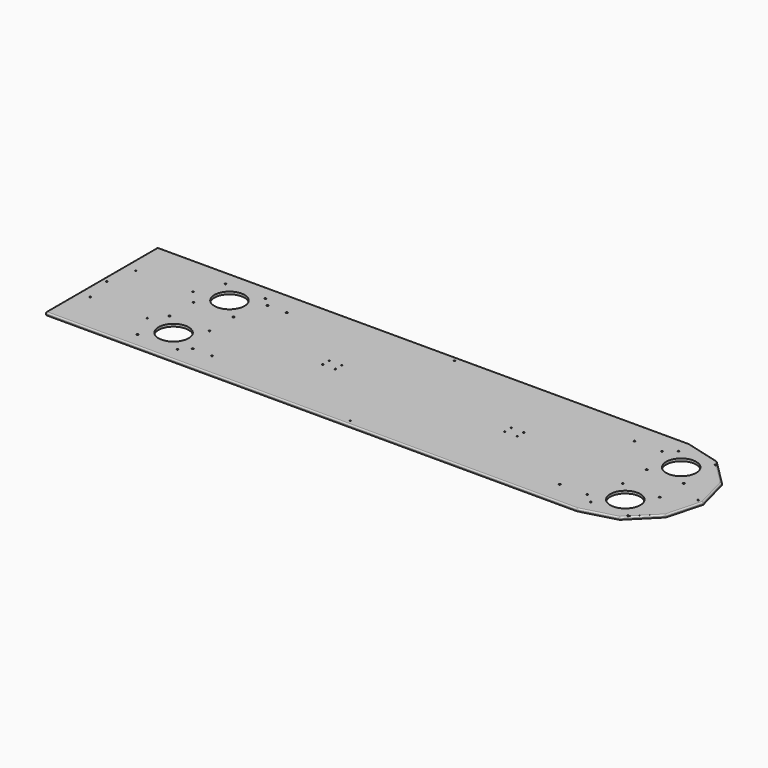
from build123d import *

# Parameters (mm, degrees)
F0_R         = 1.7272
F1_DEPTH     = 6.35
F2_R         = 1.7272
F2_R_2       = 38.1
F2_R_3       = 2.15265
F3_DEPTH     = 6.35
F4_R         = 1.7272
F4_R_2       = 2.15265
F5_DEPTH     = 6.35
F6_R         = 3.96875
F7_T1_DEPTH  = 90.4501332312
F7_T3_DEPTH  = 89.9092057235
F7_T5_DEPTH  = 1341.7087541502
F7_T7_DEPTH  = 89.9092057235
F7_T9_DEPTH  = 347.6625
F7_T11_DEPTH = 89.9092057235
F7_T13_DEPTH = 89.9092057235
F7_T15_DEPTH = 90.4501332312
F7_T18_ANGLE = 90
F7_T20_ANGLE = 30
F7_T22_ANGLE = 15
F7_T24_ANGLE = 30
F7_T26_ANGLE = 90
F7_T28_ANGLE = 30
F7_T30_ANGLE = 30
F7_T32_ANGLE = 15
F7_T34_ANGLE = 30


# Not quite as in the source:
# - a fillet or chamfer that OpenCascade refuses, or shapes differently, is made with other operations: its cross-section is extruded or revolved along the edge and cut away or added


with BuildPart() as f1:
    # F0 (on Top) → F1 (new body)
    with BuildSketch(Plane.XY):
        Polygon((88.9, 153.9793167929), (0, 177.8), (-1346.2, 177.8), (-1346.2, -177.8), (0, -177.8), (88.9, -153.9793167929), (153.9793167929, -88.9), (177.8, 0), (153.9793167929, 88.9), align=None)
        with Locations((-1316.83125, -72.23125)):
            Circle(F0_R, mode=Mode.SUBTRACT)
        with Locations((-1172.36875, -72.23125)):
            Circle(F0_R, mode=Mode.SUBTRACT)
        with Locations((-1316.83125, 72.23125)):
            Circle(F0_R, mode=Mode.SUBTRACT)
        with Locations((-1172.36875, 72.23125)):
            Circle(F0_R, mode=Mode.SUBTRACT)
    extrude(amount=F1_DEPTH)

    # F2 (on face) → F3 (cut, through all)
    with BuildSketch(Plane.XY.offset(6.35)):
        with Locations((-1333.0519925088, 0)):
            Circle(F2_R)
        with Locations((-584.2, 164.6519925088)):
            Circle(F2_R)
        with Locations((-584.2, -164.6519925088)):
            Circle(F2_R)
        with Locations((164.6519925088, 0)):
            Circle(F2_R)
        with Locations((51.0994784628, 88.5068929378)):
            Circle(F2_R_2)
        with Locations((51.0994784628, -88.5068929378)):
            Circle(F2_R_2)
        with Locations((-1092.835, 88.5068929378)):
            Circle(F2_R_2)
        with Locations((-1092.835, -88.5068929378)):
            Circle(F2_R_2)
        with Locations((4.1340214009, -139.1330868203)):
            Circle(F2_R_3)
        with Locations((98.0649355247, -139.1330868203)):
            Circle(F2_R_3)
        with Locations((98.0649355247, -37.8806990553)):
            Circle(F2_R_3)
        with Locations((4.1340214009, -37.8806990553)):
            Circle(F2_R_3)
        with Locations((4.1340214009, 37.8806990553)):
            Circle(F2_R_3)
        with Locations((4.1340214009, 139.1330868203)):
            Circle(F2_R_3)
        with Locations((98.0649355247, 139.1330868203)):
            Circle(F2_R_3)
        with Locations((98.0649355247, 37.8806990553)):
            Circle(F2_R_3)
        with Locations((-1143.4611938825, -139.1330868203)):
            Circle(F2_R_3)
        with Locations((-1042.2088061175, -139.1330868203)):
            Circle(F2_R_3)
        with Locations((-1042.2088061175, -37.8806990553)):
            Circle(F2_R_3)
        with Locations((-1143.4611938825, -37.8806990553)):
            Circle(F2_R_3)
        with Locations((-1143.4611938825, 37.8806990553)):
            Circle(F2_R_3)
        with Locations((-1042.2088061175, 37.8806990553)):
            Circle(F2_R_3)
        with Locations((-1042.2088061175, 139.1330868203)):
            Circle(F2_R_3)
        with Locations((-1143.4611938825, 139.1330868203)):
            Circle(F2_R_3)
    extrude(amount=-F3_DEPTH, mode=Mode.SUBTRACT)

    # F4 (on face) → F5 (cut, through all)
    with BuildSketch(Plane.XY.offset(6.35)):
        with Locations((-285.3053159686, -10.31875)):
            Circle(F4_R)
        with Locations((-317.0553159686, -10.31875)):
            Circle(F4_R)
        with Locations((-317.0553159686, 10.31875)):
            Circle(F4_R)
        with Locations((-285.3053159686, 10.31875)):
            Circle(F4_R)
        with Locations((-745.6803159686, 10.31875)):
            Circle(F4_R)
        with Locations((-745.6803159686, -10.31875)):
            Circle(F4_R)
        with Locations((-777.4303159686, -10.31875)):
            Circle(F4_R)
        with Locations((-777.4303159686, 10.31875)):
            Circle(F4_R)
        with Locations((-21.2905215372, 118.3676195)):
            Circle(F4_R_2)
        with Locations((-91.0257389372, 118.3676195)):
            Circle(F4_R_2)
        with Locations((-91.0257389372, -118.3676195)):
            Circle(F4_R_2)
        with Locations((-21.2905215372, -118.3676195)):
            Circle(F4_R_2)
        with Locations((-1020.445, -118.3676195)):
            Circle(F4_R_2)
        with Locations((-971.709893, -118.3676195)):
            Circle(F4_R_2)
        with Locations((-1020.445, 118.3676195)):
            Circle(F4_R_2)
        with Locations((-971.709893, 118.3676195)):
            Circle(F4_R_2)
    extrude(amount=-F5_DEPTH, mode=Mode.SUBTRACT)

    # F6
    f6_edges = [f1.edges().sort_by_distance(p)[0] for p in [
        (0, -177.8, 3.175),
        (88.9, -153.979317, 3.175),
        (153.979317, -88.9, 3.175),
        (177.8, 0, 3.175),
        (153.979317, 88.9, 3.175),
        (88.9, 153.979317, 3.175),
        (0, 177.8, 3.175),
        (-1346.2, 177.8, 3.175),
        (-1346.2, -177.8, 3.175),
    ]]
    fillet(f6_edges, radius=F6_R)

    # F7: fillet of radius 3.175 on 18 edges, made by hand

    # F7_s2 → F7_t1 (cut)
    with BuildSketch(Plane(origin=(43.4228119147, -11.6351073856, 0), x_dir=(0, 0, 1), z_dir=(-0.9659258263, 0.2588190451, 0))):
        with BuildLine():
            ThreePointArc((3.175, 171.7416119142), (5.4200640303, 170.8116759445), (6.35, 168.5666119142))
            Line((6.35, 168.5666119142), (6.35, 171.7416119142))
            Line((6.35, 171.7416119142), (3.175, 171.7416119142))
        make_face()
    extrude(amount=F7_T1_DEPTH, mode=Mode.SUBTRACT)

    # F7_s4 → F7_t3 (cut)
    with BuildSketch(Plane(origin=(31.7877045291, -31.7877045291, 0), x_dir=(0, 0, 1), z_dir=(-0.7071067812, 0.7071067812, 0))):
        with BuildLine():
            ThreePointArc((6.35, 168.5666119142), (5.4200640303, 170.8116759445), (3.175, 171.7416119142))
            Line((3.175, 171.7416119142), (6.35, 171.7416119142))
            Line((6.35, 171.7416119142), (6.35, 168.5666119142))
        make_face()
    extrude(amount=F7_T3_DEPTH, mode=Mode.SUBTRACT)

    # F7_s6 → F7_t5 (cut)
    with BuildSketch(Plane.YZ.offset(-1342.23125)):
        with BuildLine():
            ThreePointArc((174.625, 6.35), (176.8700640303, 5.4200640303), (177.8, 3.175))
            Line((177.8, 3.175), (177.8, 6.35))
            Line((177.8, 6.35), (174.625, 6.35))
        make_face()
        with BuildLine():
            ThreePointArc((-174.625, 6.35), (-176.8700640303, 5.4200640303), (-177.8, 3.175))
            Line((-177.8, 3.175), (-177.8, 6.35))
            Line((-177.8, 6.35), (-174.625, 6.35))
        make_face()
    extrude(amount=F7_T5_DEPTH, mode=Mode.SUBTRACT)

    # F7_s8 → F7_t7 (cut)
    with BuildSketch(Plane(origin=(11.6351073856, -43.4228119147, 0), x_dir=(0, 0, 1), z_dir=(-0.2588190451, 0.9659258263, 0))):
        with BuildLine():
            ThreePointArc((6.35, 168.5666119142), (5.4200640303, 170.8116759445), (3.175, 171.7416119142))
            Line((3.175, 171.7416119142), (6.35, 171.7416119142))
            Line((6.35, 171.7416119142), (6.35, 168.5666119142))
        make_face()
    extrude(amount=F7_T7_DEPTH, mode=Mode.SUBTRACT)

    # F7_s10 → F7_t9 (cut)
    with BuildSketch(Plane.XZ.offset(-173.83125)):
        with BuildLine():
            ThreePointArc((-1343.025, 6.35), (-1345.2700640303, 5.4200640303), (-1346.2, 3.175))
            Line((-1346.2, 3.175), (-1346.2, 6.35))
            Line((-1346.2, 6.35), (-1343.025, 6.35))
        make_face()
    extrude(amount=F7_T9_DEPTH, mode=Mode.SUBTRACT)

    # F7_s12 → F7_t11 (cut)
    with BuildSketch(Plane(origin=(-11.6351073856, -43.4228119147, 0), x_dir=(0, 0, 1), z_dir=(0.2588190451, 0.9659258263, 0))):
        with BuildLine():
            ThreePointArc((6.35, 168.5666119142), (5.4200640303, 170.8116759445), (3.175, 171.7416119142))
            Line((3.175, 171.7416119142), (6.35, 171.7416119142))
            Line((6.35, 171.7416119142), (6.35, 168.5666119142))
        make_face()
    extrude(amount=F7_T11_DEPTH, mode=Mode.SUBTRACT)

    # F7_s14 → F7_t13 (cut)
    with BuildSketch(Plane(origin=(-31.7877045291, -31.7877045291, 0), x_dir=(0, 0, 1), z_dir=(0.7071067812, 0.7071067812, 0))):
        with BuildLine():
            ThreePointArc((6.35, 168.5666119142), (5.4200640303, 170.8116759445), (3.175, 171.7416119142))
            Line((3.175, 171.7416119142), (6.35, 171.7416119142))
            Line((6.35, 171.7416119142), (6.35, 168.5666119142))
        make_face()
    extrude(amount=F7_T13_DEPTH, mode=Mode.SUBTRACT)

    # F7_s16 → F7_t15 (cut)
    with BuildSketch(Plane(origin=(-43.9453077645, -11.7751097266, 0), x_dir=(0, 0, 1), z_dir=(0.9659258263, 0.2588190451, 0))):
        with BuildLine():
            ThreePointArc((6.35, 168.5666119142), (5.4200640303, 170.8116759445), (3.175, 171.7416119142))
            Line((3.175, 171.7416119142), (6.35, 171.7416119142))
            Line((6.35, 171.7416119142), (6.35, 168.5666119142))
        make_face()
    extrude(amount=F7_T15_DEPTH, mode=Mode.SUBTRACT)

    # F7_s17 → F7_t18 (revolve, cut)
    with BuildSketch(Plane.XZ.offset(173.83125)):
        with BuildLine():
            ThreePointArc((-1343.025, 6.35), (-1345.2700640303, 5.4200640303), (-1346.2, 3.175))
            Line((-1346.2, 3.175), (-1346.2, 6.35))
            Line((-1346.2, 6.35), (-1343.025, 6.35))
        make_face()
    revolve(axis=Axis((-1342.23125, -173.83125, 6.35), (0, 0, 1)), revolution_arc=F7_T18_ANGLE, mode=Mode.SUBTRACT)

    # F7_s19 → F7_t20 (revolve, cut)
    with BuildSketch(Plane(origin=(43.4228119147, -11.6351073856, 0), x_dir=(0, 0, 1), z_dir=(-0.9659258263, 0.2588190451, 0))):
        with BuildLine():
            ThreePointArc((3.175, 171.7416119142), (5.4200640303, 170.8116759445), (6.35, 168.5666119142))
            Line((6.35, 168.5666119142), (6.35, 171.7416119142))
            Line((6.35, 171.7416119142), (3.175, 171.7416119142))
        make_face()
    revolve(axis=Axis((86.8456238295, 150.4210328877, 6.35), (0, 0, -1)), revolution_arc=F7_T20_ANGLE, mode=Mode.SUBTRACT)

    # F7_s21 → F7_t22 (revolve, cut)
    with BuildSketch(Plane(origin=(-43.9453077646, 11.7751097266, 0), x_dir=(0, 0, 1), z_dir=(0.9659258263, -0.2588190451, 0))):
        with BuildLine():
            ThreePointArc((3.175, -171.7416119142), (5.4200640303, -170.8116759445), (6.35, -168.5666119142))
            Line((6.35, -168.5666119142), (6.35, -171.7416119142))
            Line((6.35, -171.7416119142), (3.175, -171.7416119142))
        make_face()
    revolve(axis=Axis((-0.5224958498, 173.83125, 6.35), (0, 0, 1)), revolution_arc=F7_T22_ANGLE, mode=Mode.SUBTRACT)

    # F7_s23 → F7_t24 (revolve, cut)
    with BuildSketch(Plane(origin=(31.7877045291, -31.7877045291, 0), x_dir=(0, 0, 1), z_dir=(-0.7071067812, 0.7071067812, 0))):
        with BuildLine():
            ThreePointArc((6.35, 168.5666119142), (5.4200640303, 170.8116759445), (3.175, 171.7416119142))
            Line((3.175, 171.7416119142), (6.35, 171.7416119142))
            Line((6.35, 171.7416119142), (6.35, 168.5666119142))
        make_face()
    revolve(axis=Axis((150.4210328877, 86.8456238295, 6.35), (0, 0, -1)), revolution_arc=F7_T24_ANGLE, mode=Mode.SUBTRACT)

    # F7_s25 → F7_t26 (revolve, cut)
    with BuildSketch(Plane.YZ.offset(-1342.23125)):
        with BuildLine():
            ThreePointArc((174.625, 6.35), (176.8700640303, 5.4200640303), (177.8, 3.175))
            Line((177.8, 3.175), (177.8, 6.35))
            Line((177.8, 6.35), (174.625, 6.35))
        make_face()
    revolve(axis=Axis((-1342.23125, 173.83125, 6.35), (0, 0, 1)), revolution_arc=F7_T26_ANGLE, mode=Mode.SUBTRACT)

    # F7_s27 → F7_t28 (revolve, cut)
    with BuildSketch(Plane(origin=(11.6351073856, -43.4228119147, 0), x_dir=(0, 0, 1), z_dir=(-0.2588190451, 0.9659258263, 0))):
        with BuildLine():
            ThreePointArc((6.35, 168.5666119142), (5.4200640303, 170.8116759445), (3.175, 171.7416119142))
            Line((3.175, 171.7416119142), (6.35, 171.7416119142))
            Line((6.35, 171.7416119142), (6.35, 168.5666119142))
        make_face()
    revolve(axis=Axis((173.691247659, 0, 6.35), (0, 0, -1)), revolution_arc=F7_T28_ANGLE, mode=Mode.SUBTRACT)

    # F7_s29 → F7_t30 (revolve, cut)
    with BuildSketch(Plane(origin=(-11.6351073856, -43.4228119147, 0), x_dir=(0, 0, 1), z_dir=(0.2588190451, 0.9659258263, 0))):
        with BuildLine():
            ThreePointArc((6.35, 168.5666119142), (5.4200640303, 170.8116759445), (3.175, 171.7416119142))
            Line((3.175, 171.7416119142), (6.35, 171.7416119142))
            Line((6.35, 171.7416119142), (6.35, 168.5666119142))
        make_face()
    revolve(axis=Axis((150.4210328877, -86.8456238295, 6.35), (0, 0, -1)), revolution_arc=F7_T30_ANGLE, mode=Mode.SUBTRACT)

    # F7_s31 → F7_t32 (revolve, cut)
    with BuildSketch(Plane.YZ.offset(-0.5224958498)):
        with BuildLine():
            ThreePointArc((-174.625, 6.35), (-176.8700640303, 5.4200640303), (-177.8, 3.175))
            Line((-177.8, 3.175), (-177.8, 6.35))
            Line((-177.8, 6.35), (-174.625, 6.35))
        make_face()
    revolve(axis=Axis((-0.5224958498, -173.83125, 6.35), (0, 0, 1)), revolution_arc=F7_T32_ANGLE, mode=Mode.SUBTRACT)

    # F7_s33 → F7_t34 (revolve, cut)
    with BuildSketch(Plane(origin=(-31.7877045291, -31.7877045291, 0), x_dir=(0, 0, 1), z_dir=(0.7071067812, 0.7071067812, 0))):
        with BuildLine():
            ThreePointArc((6.35, 168.5666119142), (5.4200640303, 170.8116759445), (3.175, 171.7416119142))
            Line((3.175, 171.7416119142), (6.35, 171.7416119142))
            Line((6.35, 171.7416119142), (6.35, 168.5666119142))
        make_face()
    revolve(axis=Axis((86.8456238295, -150.4210328877, 6.35), (0, 0, -1)), revolution_arc=F7_T34_ANGLE, mode=Mode.SUBTRACT)


solid = f1.part
